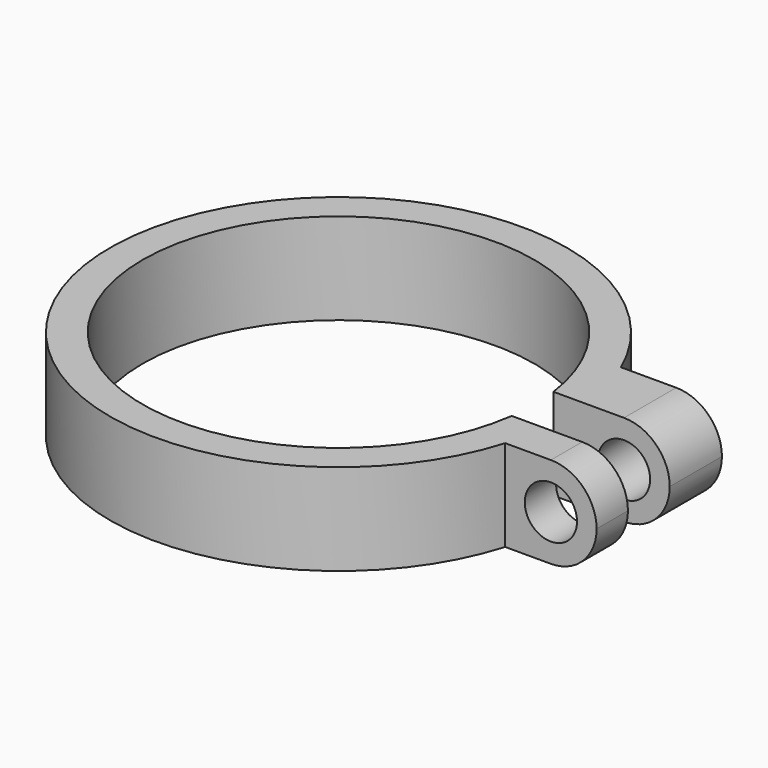
from build123d import *

# Parameters (mm, degrees)
F0_W     = 7
F0_H     = 2
F1_DEPTH = 7
F2_R     = 2
F3_DEPTH = 25
F4_R     = 3.49999


# Not quite as in the source:
# - a fillet or chamfer is up to 0.001 mm smaller than in the source, because OpenCascade refuses the exact size


with BuildPart() as f1:
    # F0 (on Top) → F1 (new body)
    with BuildSketch(Plane.XY):
        with BuildLine():
            ThreePointArc((14.8660687473, -2), (-15, 0), (14.8660687473, 2))
            Line((14.8660687473, 2), (16.7705098312, 2))
            Line((16.7705098312, 2), (16.7705098312, 5))
            Line((16.7705098312, 5), (16.0390149323, 5))
            Line((16.0390149323, 5), (16.0390149323, 7))
            ThreePointArc((16.0390149323, 7), (-17.4675765006, -1.0647869255), (16.7705098312, -5))
            Line((16.7705098312, -5), (16.7705098312, -2))
            Line((16.7705098312, -2), (14.8660687473, -2))
        make_face()
        with BuildLine():
            Line((16.7705098312, 5), (16.7705098312, 2))
            Line((16.7705098312, 2), (17.3853386507, 2))
            ThreePointArc((17.3853386507, 2), (17.1436721965, 3.5134745793), (16.7705098312, 5))
        make_face()
        with BuildLine():
            ThreePointArc((16.7705098312, 5), (17.1436721965, 3.5134745793), (17.3853386507, 2))
            Line((17.3853386507, 2), (23.7705098312, 2))
            Line((23.7705098312, 2), (23.7705098312, 5))
            Line((23.7705098312, 5), (16.7705098312, 5))
        make_face()
        with BuildLine():
            Line((23.7705098312, -2), (17.3853386507, -2))
            ThreePointArc((17.3853386507, -2), (17.1436721965, -3.5134745793), (16.7705098312, -5))
            Line((16.7705098312, -5), (23.7705098312, -5))
            Line((23.7705098312, -5), (23.7705098312, -2))
        make_face()
        with BuildLine():
            Line((17.3853386507, -2), (16.7705098312, -2))
            Line((16.7705098312, -2), (16.7705098312, -5))
            ThreePointArc((16.7705098312, -5), (17.1436721965, -3.5134745793), (17.3853386507, -2))
        make_face()
        with Locations((20.2705098312, 6)):
            Rectangle(F0_W, F0_H)
        with BuildLine():
            Line((16.0390149323, 5), (16.7705098312, 5))
            ThreePointArc((16.7705098312, 5), (16.4352130745, 6.0111372632), (16.0390149323, 7))
            Line((16.0390149323, 7), (16.0390149323, 5))
        make_face()
        with BuildLine():
            ThreePointArc((16.0390149323, 7), (16.4352130745, 6.0111372632), (16.7705098312, 5))
            Line((16.7705098312, 5), (16.7705098312, 7))
            Line((16.7705098312, 7), (16.0390149323, 7))
        make_face()
    extrude(amount=F1_DEPTH)

    # F2 (on face) → F3 (cut)
    with BuildSketch(Plane.XZ.offset(5)):
        with Locations((20.2705098312, 3.5)):
            Circle(F2_R)
    extrude(amount=-F3_DEPTH, mode=Mode.SUBTRACT)

    # F4 (radius 3.5 in the source; OpenCascade refuses exactly that, so slightly less here)
    f4_edges = [f1.edges().sort_by_distance(p)[0] for p in [
        (23.77051, -3.5, 7),
        (23.77051, 4.5, 7),
        (23.77051, -3.5, 0),
        (23.77051, 4.5, 0),
    ]]
    fillet(f4_edges, radius=F4_R)


solid = f1.part
